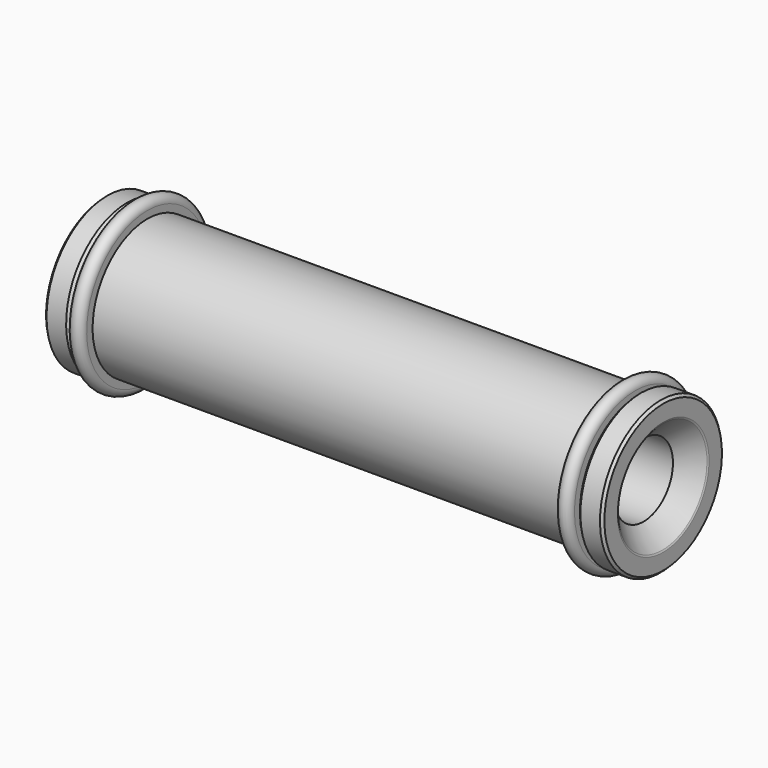
from build123d import *

# Parameters (mm, degrees)
F2_SIZE = 4


# Not quite as in the source:
# - a fillet or chamfer that OpenCascade refuses, or shapes differently, is made with other operations: its cross-section is extruded or revolved along the edge and cut away or added


with BuildPart() as f1:
    # F0 (on Front) → F1 (revolve)
    with BuildSketch(Plane.XZ):
        with BuildLine():
            Line((-55, 0), (-55, 7.5))
            Line((-55, 7.5), (55, 7.5))
            Line((55, 7.5), (55, 15.5))
            Line((55, 15.5), (50, 15.5))
            Line((50, 15.5), (50, 13.5))
            Line((50, 13.5), (49.3, 13.5))
            Line((49.3, 13.5), (49.3, 15.5))
            ThreePointArc((49.3, 15.5), (47.8, 17), (46.3, 15.5))
            Line((46.3, 15.5), (46.3, 14))
            Line((46.3, 14), (-50.3, 14))
            Line((-50.3, 14), (-50.3, 15.5))
            ThreePointArc((-50.3, 15.5), (-51.8, 17.0770088649), (-53.3, 15.5))
            Line((-53.3, 15.5), (-53.3, 13.5))
            Line((-53.3, 13.5), (-54, 13.5))
            Line((-54, 13.5), (-54, 15.5))
            Line((-54, 15.5), (-59, 15.5))
            Line((-59, 15.5), (-59, 0))
            Line((-59, 0), (-55, 0))
        make_face()
    revolve(axis=Axis((-4.5135766268, 0, 0), (1, 0, 0)))

    # F2
    f2_edges = [f1.edges().sort_by_distance(p)[0] for p in [
        (55, 0, -7.5),
    ]]
    chamfer(f2_edges, length=F2_SIZE)

    # F3: chamfer of 0.5 on 5 edges, made by hand

    # F3_s1 → F3_t2 (revolve, cut)
    with BuildSketch(Plane.XZ):
        Polygon((55, 15), (54.5, 15.5), (55, 15.5), align=None)
    revolve(axis=Axis((55, 0, 0), (1, 0, 0)), mode=Mode.SUBTRACT)

    # F3_s3 → F3_t4 (revolve, cut)
    with BuildSketch(Plane.XZ):
        Polygon((54.8535533906, 11.3535533906), (55, 11.7071067812), (55, 11.5), align=None)
    revolve(axis=Axis((55, 0, 0), (1, 0, 0)), mode=Mode.SUBTRACT)

    # F3_s5 → F3_t6 (revolve, cut)
    with BuildSketch(Plane.XZ):
        Polygon((-58.5, 15.5), (-59, 15), (-59, 15.5), align=None)
    revolve(axis=Axis((-59, 0, 0), (1, 0, 0)), mode=Mode.SUBTRACT)

    # F3_s7 → F3_t8 (revolve, cut)
    with BuildSketch(Plane.XZ):
        Polygon((-54, 15), (-54.5, 15.5), (-54, 15.5), align=None)
    revolve(axis=Axis((-54, 0, 0), (1, 0, 0)), mode=Mode.SUBTRACT)

    # F3_s9 → F3_t10 (revolve, cut)
    with BuildSketch(Plane.XZ):
        Polygon((50.5, 15.5), (50, 15), (50, 15.5), align=None)
    revolve(axis=Axis((50, 0, 0), (1, 0, 0)), mode=Mode.SUBTRACT)


solid = f1.part
